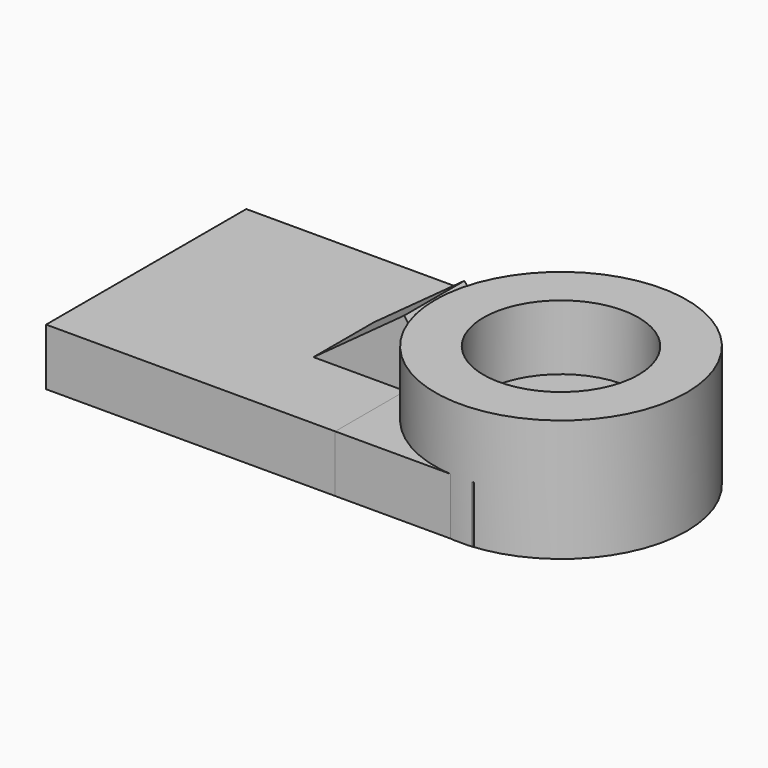
from build123d import *

# Parameters (mm, degrees)
F0_R     = 50.0122703422
F0_R_2   = 30.8528794084
F1_DEPTH = 48.514
F2_W     = 115.0430589914
F2_H     = 22.641453892
F3_DEPTH = 49.784
F4_DEPTH = 55.118
F6_E3_W  = 44.6751625542
F6_E3_H  = 29.972
F7_DEPTH = 27.686


with BuildPart() as f1:
    # F0 (on Top) → F1 (new body)
    with BuildSketch(Plane.XY):
        Circle(F0_R)
        Circle(F0_R_2, mode=Mode.SUBTRACT)
    extrude(amount=F1_DEPTH)


with BuildPart() as f3:
    # F2 (on Front) → F3 (new body, symmetric)
    with BuildSketch(Plane.XZ):
        with Locations((-107.546903193, 11.320726946)):
            Rectangle(F2_W, F2_H)
    extrude(amount=F3_DEPTH, both=True)


with BuildPart() as f4:
    # F4 (new): a face of the model
    f4_faces = [f3.part.faces().sort_by_distance(p)[0] for p in [
        (-50.0253736973, 0, 11.320726946),
    ]]
    extrude(f4_faces, amount=F4_DEPTH)


with BuildPart() as f7:
    # F6_E3 (on explicit) → F7 (new body)
    with BuildSketch(Plane(origin=(-50.4005476832, 14.986, 48.9544942975), x_dir=(-0.8081433169, 0, -0.5889858906), z_dir=(-0.5889858906, 0, 0.8081433169))):
        with Locations((22.3375812771, 14.986)):
            Rectangle(F6_E3_W, F6_E3_H)
    extrude(amount=-F7_DEPTH)


solid = Compound([f1.part, f3.part, f4.part, f7.part])
